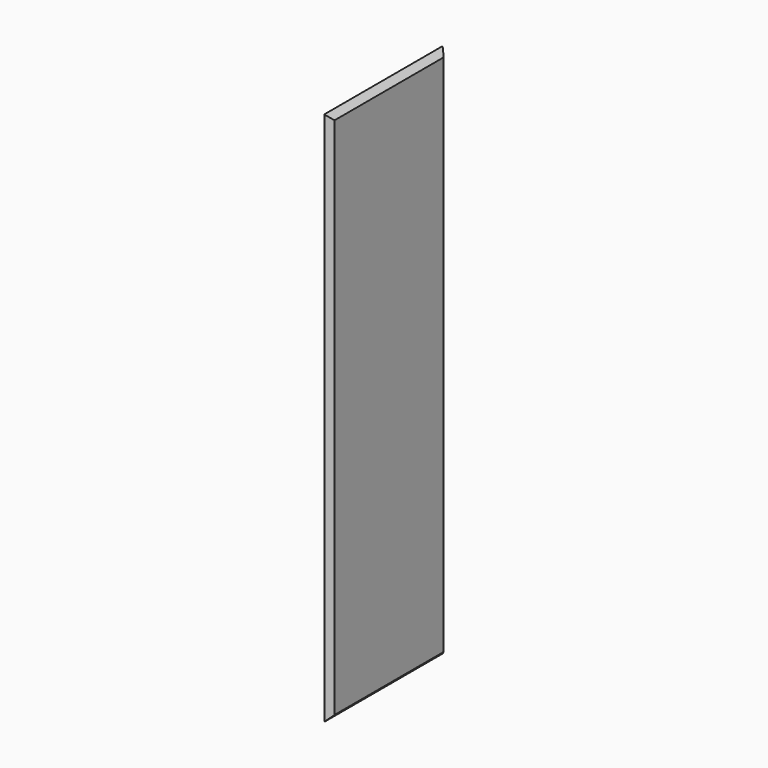
from build123d import *

# Parameters (mm, degrees)
F0_W     = 260
F0_H     = 940
F1_DEPTH = 5
F2_SIZE  = 9.99999


# Not quite as in the source:
# - a fillet or chamfer is up to 0.001 mm smaller than in the source, because OpenCascade refuses the exact size


with BuildPart() as f1:
    # F0 (on Right) → F1 (new body, symmetric)
    with BuildSketch(Plane.YZ):
        with Locations((130, -470)):
            Rectangle(F0_W, F0_H)
    extrude(amount=F1_DEPTH, both=True)

    # F2 (size 10 in the source; OpenCascade refuses exactly that, so slightly less here)
    f2_edges = [f1.edges().sort_by_distance(p)[0] for p in [
        (5, 0, -470),
        (5, 130, 0),
        (5, 260, -470),
        (5, 130, -940),
    ]]
    chamfer(f2_edges, length=F2_SIZE)


solid = f1.part
